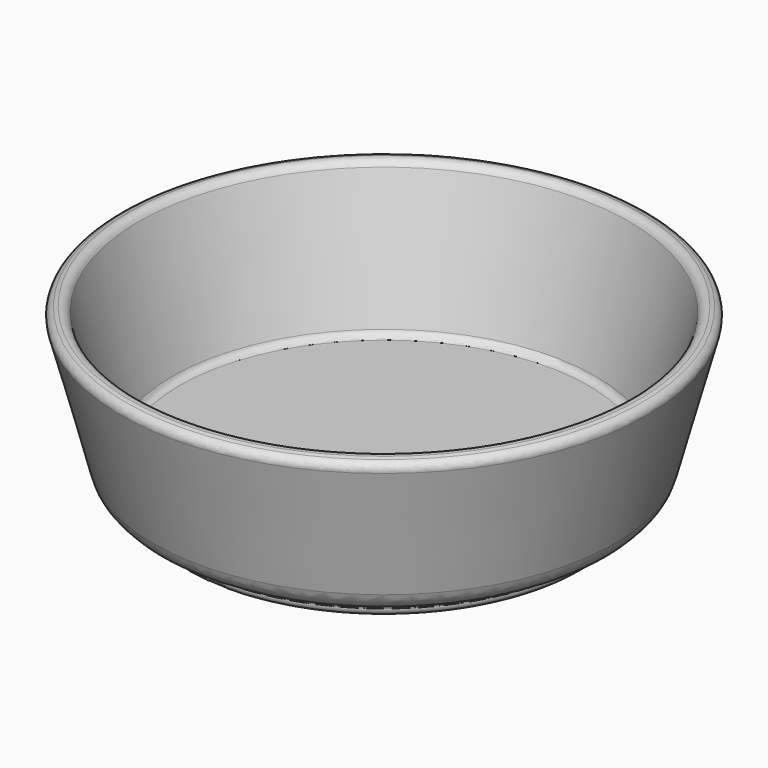
from build123d import *

# Parameters (mm, degrees)
F2_R = 3.99999
F3_R = 15


# Not quite as in the source:
# - a fillet or chamfer is up to 0.001 mm smaller than in the source, because OpenCascade refuses the exact size


with BuildPart() as f1:
    # F0 (on Front) → F1 (revolve)
    with BuildSketch(Plane.XZ):
        Polygon((-90, 0), (0, 0), (0, 10), (-110, 10), (-129.4114283827, 82.4444369717), (-139.0706866456, 79.8562465207), (-117.6732698798, 0), (-104, 0), (-104, -8), (-90, -8), align=None)
    revolve(axis=Axis((0, 0, 5), (0, 0, -1)))

    # F2 (radius 4 in the source; OpenCascade refuses exactly that, so slightly less here)
    f2_edges = [f1.edges().sort_by_distance(p)[0] for p in [
        (110, 0, 10),
        (129.411428, 0, 82.444437),
        (139.070687, 0, 79.856247),
        (104, 0, -8),
        (90, 0, -8),
        (104, 0, 0),
    ]]
    fillet(f2_edges, radius=F2_R)

    # F3
    f3_edges = [f1.edges().sort_by_distance(p)[0] for p in [
        (90, 0, 0),
        (117.67327, 0, 0),
    ]]
    fillet(f3_edges, radius=F3_R)


solid = f1.part
